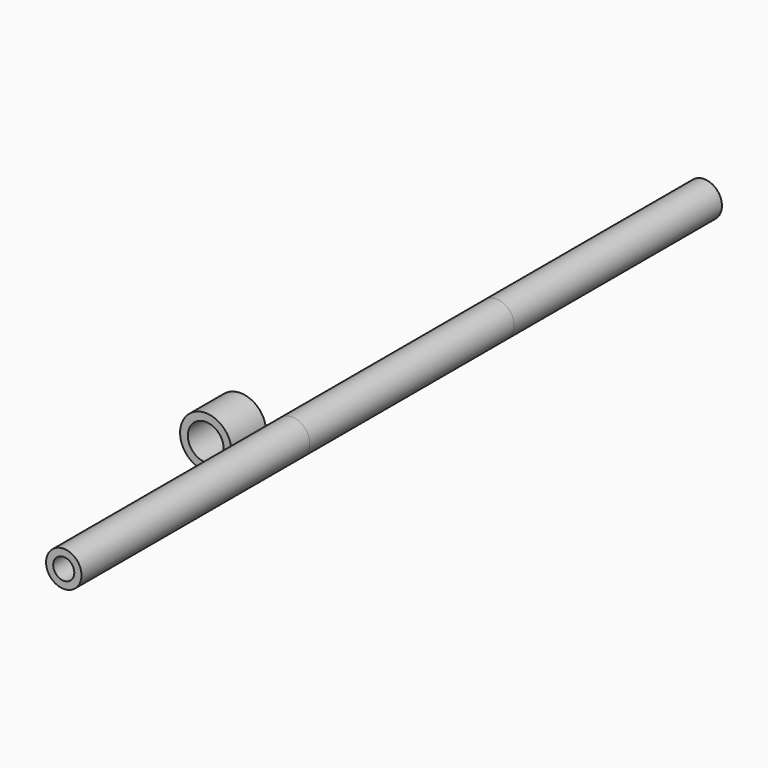
from build123d import *

# Parameters (mm, degrees)
F0_R     = 28.8966469819
F0_R_2   = 20.1306031815
F1_DEPTH = 48.768
F2_R     = 19.9266814882
F2_R_2   = 11.8595015416
F3_DEPTH = 155.194
F4_DEPTH = 165.862
F5_DEPTH = 287.528
F6_DEPTH = 292.1


with BuildPart() as f1:
    # F0 (on Front) → F1 (new body)
    with BuildSketch(Plane.XZ):
        with Locations((-39.2948538065, 30.2996449172)):
            Circle(F0_R)
        with Locations((-39.2948538065, 30.2996449172)):
            Circle(F0_R_2, mode=Mode.SUBTRACT)
    extrude(amount=F1_DEPTH)


with BuildPart() as f3:
    # F2 (on Front) → F3 (new body)
    with BuildSketch(Plane.XZ):
        with Locations((18.7794677913, 34.4027206302)):
            Circle(F2_R)
        with Locations((18.7794677913, 34.4027206302)):
            Circle(F2_R_2, mode=Mode.SUBTRACT)
    extrude(amount=F3_DEPTH)

    # F4 (add): a face of the model
    f4_faces = [f3.faces().sort_by_distance(p)[0] for p in [
        (-0.5836020326, -155.194, 34.4027206302),
    ]]
    extrude(f4_faces, amount=F4_DEPTH)

    # F5 (add): a face of the model
    f5_faces = [f3.faces().sort_by_distance(p)[0] for p in [
        (-0.5836020326, 0, 34.4027206302),
    ]]
    extrude(f5_faces, amount=F5_DEPTH)

    # F6 (add): a face of the model
    f6_faces = [f3.faces().sort_by_distance(p)[0] for p in [
        (-0.5836020326, 287.528, 34.4027206302),
    ]]
    extrude(f6_faces, amount=F6_DEPTH)


solid = Compound([f1.part, f3.part])
